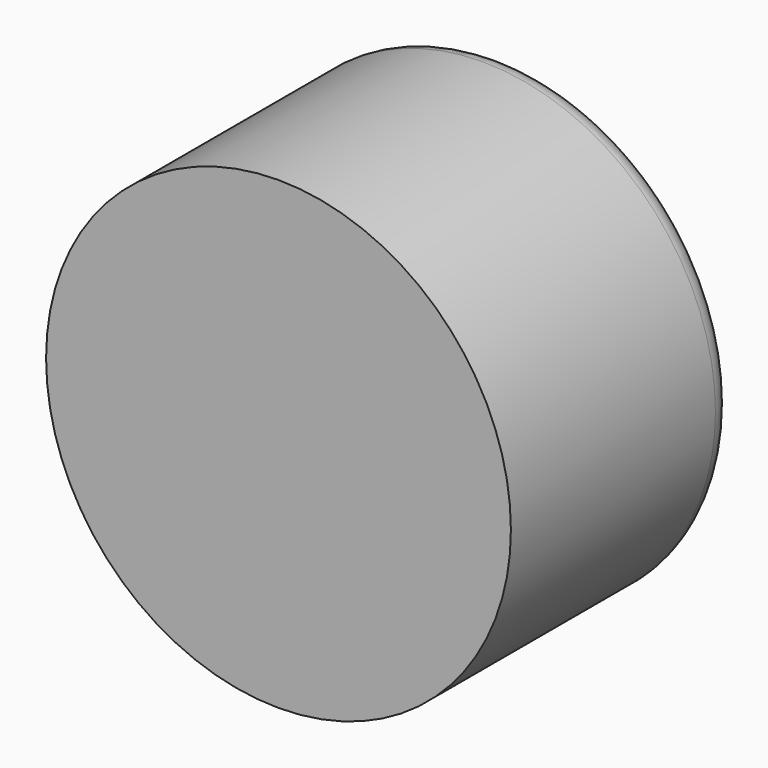
from build123d import *

# Parameters (mm, degrees)
F0_R     = 63.5
F1_DEPTH = 76.2
F2_T     = -12.7
F3_R     = 6.34999


# Not quite as in the source:
# - a fillet or chamfer is up to 0.001 mm smaller than in the source, because OpenCascade refuses the exact size


with BuildPart() as f1:
    # F0 (on Front) → F1 (new body)
    with BuildSketch(Plane.XZ):
        Circle(F0_R)
    extrude(amount=F1_DEPTH)

    # F2
    f2_openings = [f1.faces().sort_by_distance(p)[0] for p in [
        (0, 0, 0),
    ]]
    offset(amount=F2_T, openings=f2_openings)

    # F3 (radius 6.35 in the source; OpenCascade refuses exactly that, so slightly less here)
    f3_edges = [f1.edges().sort_by_distance(p)[0] for p in [
        (-63.5, 0, 0),
        (-50.8, 0, 0),
    ]]
    fillet(f3_edges, radius=F3_R)


solid = f1.part
